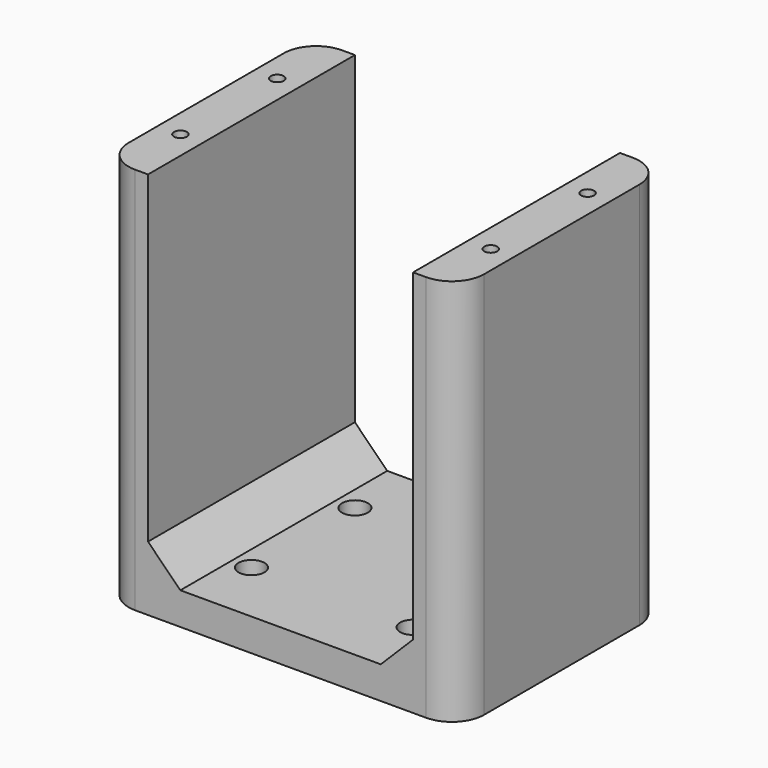
from build123d import *

# Parameters (mm, degrees)
F0_W     = 55
F0_H     = 40
F0_R     = 2
F1_DEPTH = 5
F2_W     = 7
F2_H     = 40
F3_DEPTH = 55
F4_R     = 1
F5_DEPTH = 15
F6_R     = 5
F7_W     = 5
F7_H     = 5
F8_DEPTH = 40
F9_SIZE  = 4.99999


# Not quite as in the source:
# - a fillet or chamfer is up to 0.001 mm smaller than in the source, because OpenCascade refuses the exact size


with BuildPart() as f1:
    # F0 (on Top) → F1 (new body)
    with BuildSketch(Plane.XY):
        Rectangle(F0_W, F0_H)
        with Locations((-12.5, -10)):
            Circle(F0_R, mode=Mode.SUBTRACT)
        with Locations((12.5, -10)):
            Circle(F0_R, mode=Mode.SUBTRACT)
        with Locations((-12.5, 10)):
            Circle(F0_R, mode=Mode.SUBTRACT)
        with Locations((12.5, 10)):
            Circle(F0_R, mode=Mode.SUBTRACT)
    extrude(amount=F1_DEPTH)

    # F2 (on face) → F3 (join)
    with BuildSketch(Plane.XY.offset(5)):
        with Locations((-24, 0)):
            Rectangle(F2_W, F2_H)
        with Locations((24, 0)):
            Rectangle(F2_W, F2_H)
    extrude(amount=F3_DEPTH)

    # F4 (on face) → F5 (cut)
    with BuildSketch(Plane.XY.offset(60)):
        with Locations((-24, 9.358282201)):
            Circle(F4_R)
        with Locations((24, 9.358282201)):
            Circle(F4_R)
        with Locations((24, -9.358282201)):
            Circle(F4_R)
        with Locations((-24, -9.358282201)):
            Circle(F4_R)
    extrude(amount=-F5_DEPTH, mode=Mode.SUBTRACT)

    # F6
    f6_edges = [f1.edges().sort_by_distance(p)[0] for p in [
        (-27.5, 20, 30),
        (-27.5, -20, 30),
        (27.5, -20, 30),
        (27.5, 20, 30),
    ]]
    fillet(f6_edges, radius=F6_R)

    # F7 (on face) → F8 (join)
    with BuildSketch(Plane(origin=(0, 20, 0), x_dir=(-1, 0, 0), z_dir=(0, 1, 0))):
        with Locations((-18, 7.5)):
            Rectangle(F7_W, F7_H)
        with Locations((18, 7.5)):
            Rectangle(F7_W, F7_H)
    extrude(amount=-F8_DEPTH)

    # F9 (size 5 in the source; OpenCascade refuses exactly that, so slightly less here)
    f9_edges = [f1.edges().sort_by_distance(p)[0] for p in [
        (15.5, 0, 10),
        (-15.5, 0, 10),
    ]]
    chamfer(f9_edges, length=F9_SIZE)


solid = f1.part
